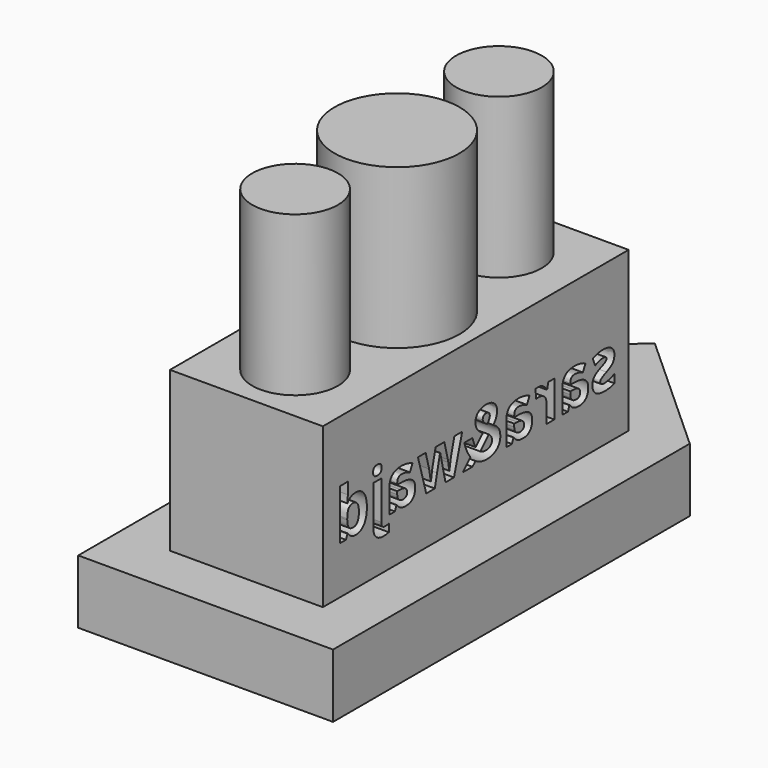
from build123d import *

# Parameters (mm, degrees)
F1_DEPTH     = 10
F2_W         = 24
F2_H         = 60
F3_DEPTH     = 25
F4_R         = 6.7288508224
F4_R_2       = 9.8144467468
F5_DEPTH     = 25
F6_TEXT_SIZE = 10.388383898
F7_DEPTH     = 25


# Not quite as in the source:
# - Text() gives the source's letters only with a copy of the font that has no kerning and outlines rounded to 1/6400 em; it was checked with that copy


with BuildPart() as f1:
    # F0 (on Top) → F1 (new body)
    with BuildSketch(Plane.XY):
        Polygon((0, 50.581280164), (-20, 32.4429230167), (-20, -37.5570769833), (20, -37.5570769833), (20, 32.4429230167), align=None)
    extrude(amount=F1_DEPTH)

    # F2 (on face) → F3 (join)
    with BuildSketch(Plane.XY.offset(10)):
        with Locations((0, 0.4429230167)):
            Rectangle(F2_W, F2_H)
    extrude(amount=F3_DEPTH)

    # F4 (on face) → F5 (join)
    with BuildSketch(Plane.XY.offset(35)):
        with Locations((0, 20)):
            Circle(F4_R)
        Circle(F4_R_2)
        with Locations((0, -20)):
            Circle(F4_R)
    extrude(amount=F5_DEPTH)

    # F6 (on face) → F7 (cut)
    with BuildSketch(Plane(origin=(-12, 0, 0), x_dir=(0, -1, 0), z_dir=(-1, 0, 0))):
        with Locations((-28.1127272491, 17.4709784166)):
            Text('sara&wajd', F6_TEXT_SIZE, font='Open Sans', font_style=FontStyle.BOLD, text_align=(TextAlign.LEFT, TextAlign.BOTTOM))
    extrude(amount=-F7_DEPTH, mode=Mode.SUBTRACT)


solid = f1.part
